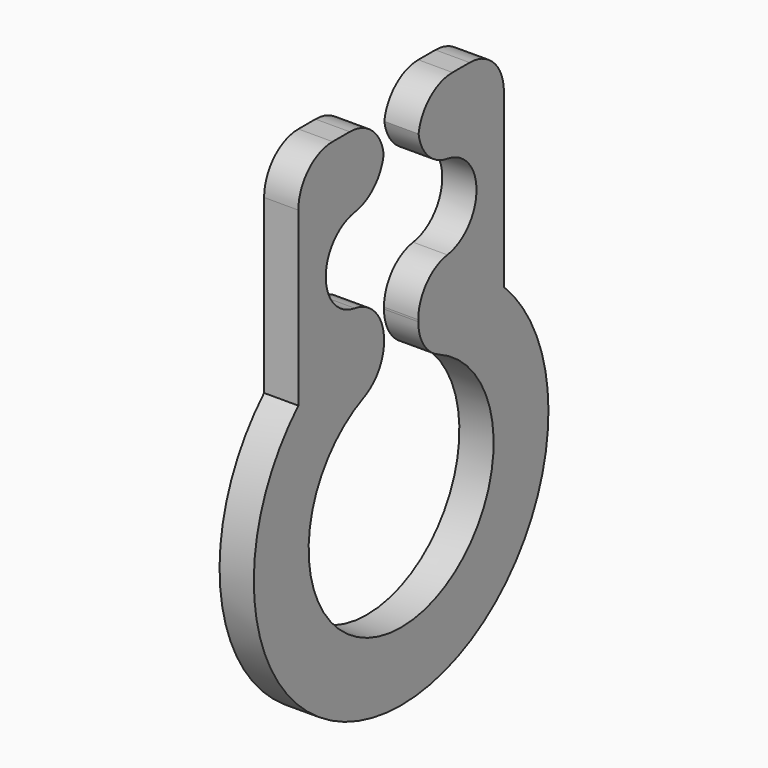
from build123d import *

# Parameters (mm, degrees)
F1_DEPTH    = 0.4
F2_T1_DEPTH = 2.9
F2_T3_DEPTH = 2.8434299833
F2_T5_DEPTH = 2.2225176819


# Not quite as in the source:
# - a fillet or chamfer that OpenCascade refuses, or shapes differently, is made with other operations: its cross-section is extruded or revolved along the edge and cut away or added


with BuildPart() as f1:
    # F0 (on Right) → F1 (new body)
    with BuildSketch(Plane.YZ):
        with BuildLine():
            ThreePointArc((0.25, 1.3266499161), (0, -1.35), (-0.25, 1.3266499161))
            Line((-0.25, 1.3266499161), (-0.25, 2.2))
            Line((-0.25, 2.2), (-0.6, 2.2))
            ThreePointArc((-0.6, 2.2), (-1.1, 2.7), (-0.6, 3.2))
            Line((-0.6, 3.2), (-0.25, 3.2))
            Line((-0.25, 3.2), (-0.25, 4.05))
            Line((-0.25, 4.05), (-1.5, 4.05))
            Line((-1.5, 4.05), (-1.5, 1.5402921801))
            ThreePointArc((-1.5, 1.5402921801), (0, -2.15), (1.5, 1.5402921801))
            Line((1.5, 1.5402921801), (1.5, 4.05))
            Line((1.5, 4.05), (0.25, 4.05))
            Line((0.25, 4.05), (0.25, 3.2))
            Line((0.25, 3.2), (0.6, 3.2))
            ThreePointArc((0.6, 3.2), (1.1, 2.7), (0.6, 2.2))
            Line((0.6, 2.2), (0.25, 2.2))
            Line((0.25, 2.2), (0.25, 1.3266499161))
        make_face()
    extrude(amount=F1_DEPTH)

    # F2: fillet of radius 0.5 on 10 edges, made by hand

    # F2_s2 → F2_t1 (cut)
    with BuildSketch(Plane.YZ.offset(-1.25)):
        with BuildLine():
            ThreePointArc((-0.25, 3.55), (-0.3964466094, 3.9035533906), (-0.75, 4.05))
            Line((-0.75, 4.05), (-0.25, 4.05))
            Line((-0.25, 4.05), (-0.25, 3.55))
        make_face()
        with BuildLine():
            ThreePointArc((-1, 4.05), (-1.3535533906, 3.9035533906), (-1.5, 3.55))
            Line((-1.5, 3.55), (-1.5, 4.05))
            Line((-1.5, 4.05), (-1, 4.05))
        make_face()
        with BuildLine():
            ThreePointArc((0.75, 4.05), (0.3964466094, 3.9035533906), (0.25, 3.55))
            Line((0.25, 3.55), (0.25, 4.05))
            Line((0.25, 4.05), (0.75, 4.05))
        make_face()
        with BuildLine():
            ThreePointArc((1.5, 3.55), (1.3535533906, 3.9035533906), (1, 4.05))
            Line((1, 4.05), (1.5, 4.05))
            Line((1.5, 4.05), (1.5, 3.55))
        make_face()
    extrude(amount=F2_T1_DEPTH, mode=Mode.SUBTRACT)

    # F2_s4 → F2_t3 (cut)
    with BuildSketch(Plane.YZ.offset(-1.2217149917)):
        with BuildLine():
            ThreePointArc((-0.675, 3.1943429983), (-0.3708562278, 3.3627258764), (-0.25, 3.6886859967))
            Line((-0.25, 3.6886859967), (-0.2, 3.6886859967))
            Line((-0.2, 3.6886859967), (-0.2, 3.2))
            Line((-0.2, 3.2), (-0.25, 3.15))
            ThreePointArc((-0.25, 3.15), (-0.6, 3.15), (-0.6675, 3.1449086985))
            Line((-0.6675, 3.1449086985), (-0.675, 3.1943429983))
        make_face()
        with BuildLine():
            ThreePointArc((-0.25, 1.7113140033), (-0.3708562278, 2.0372741236), (-0.675, 2.2056570017))
            Line((-0.675, 2.2056570017), (-0.6675, 2.2550913015))
            ThreePointArc((-0.6675, 2.2550913015), (-0.6, 2.25), (-0.25, 2.25))
            Line((-0.25, 2.25), (-0.2, 2.2))
            Line((-0.2, 2.2), (-0.2, 1.7113140033))
            Line((-0.2, 1.7113140033), (-0.25, 1.7113140033))
        make_face()
        with BuildLine():
            ThreePointArc((0.675, 2.2056570017), (0.3708562278, 2.0372741236), (0.25, 1.7113140033))
            Line((0.25, 1.7113140033), (0.2, 1.7113140033))
            Line((0.2, 1.7113140033), (0.2, 2.2))
            Line((0.2, 2.2), (0.25, 2.25))
            ThreePointArc((0.25, 2.25), (0.6, 2.25), (0.6675, 2.2550913015))
            Line((0.6675, 2.2550913015), (0.675, 2.2056570017))
        make_face()
        with BuildLine():
            ThreePointArc((0.25, 3.6886859967), (0.3708562278, 3.3627258764), (0.675, 3.1943429983))
            Line((0.675, 3.1943429983), (0.6675, 3.1449086985))
            ThreePointArc((0.6675, 3.1449086985), (0.6, 3.15), (0.25, 3.15))
            Line((0.25, 3.15), (0.2, 3.2))
            Line((0.2, 3.2), (0.2, 3.6886859967))
            Line((0.2, 3.6886859967), (0.25, 3.6886859967))
        make_face()
    extrude(amount=F2_T3_DEPTH, mode=Mode.SUBTRACT)

    # F2_s6 → F2_t5 (cut)
    with BuildSketch(Plane.YZ.offset(-0.911258841)):
        with BuildLine():
            ThreePointArc((0.25, 1.6911534525), (0.3308631779, 1.4185285741), (0.5472972973, 1.2340849518))
            ThreePointArc((0.5472972973, 1.2340849518), (0.4013263176, 1.2889674886), (0.25, 1.3266499161))
            Line((0.25, 1.3266499161), (0.25, 1.6911534525))
        make_face()
        with BuildLine():
            ThreePointArc((-0.5472972973, 1.2340849518), (-0.3308631779, 1.4185285741), (-0.25, 1.6911534525))
            Line((-0.25, 1.6911534525), (-0.25, 1.3266499161))
            ThreePointArc((-0.25, 1.3266499161), (-0.4013263176, 1.2889674886), (-0.5472972973, 1.2340849518))
        make_face()
    extrude(amount=F2_T5_DEPTH, mode=Mode.SUBTRACT)


solid = f1.part
